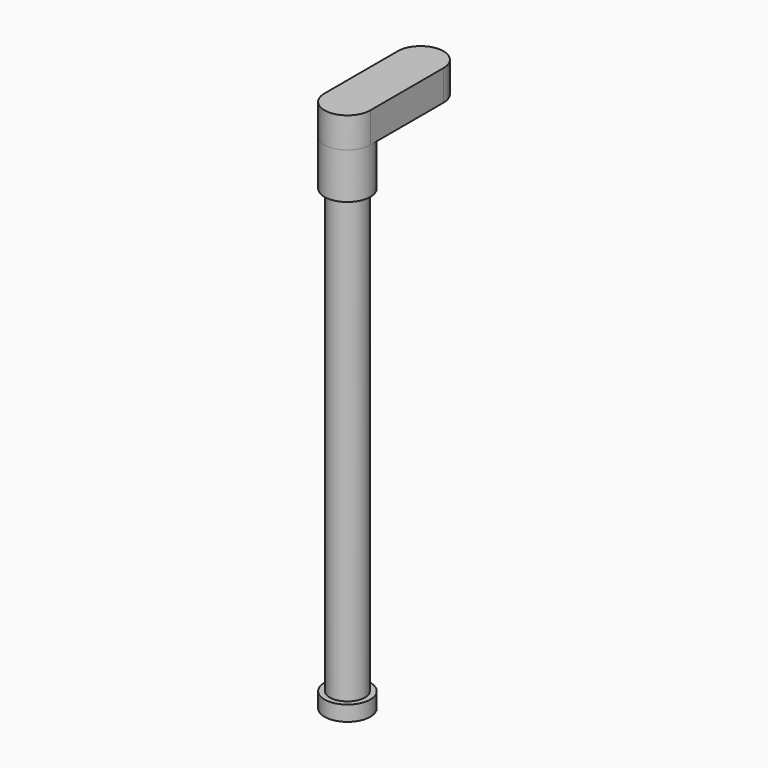
from build123d import *

# Parameters (mm, degrees)
F0_R     = 2.921
F1_DEPTH = 73.66
F2_R     = 3.81
F2_R_2   = 2.921
F3_DEPTH = 2.54
F4_R     = 3.81
F5_DEPTH = 7.62
F7_DEPTH = 5.08


with BuildPart() as f1:
    # F0 (on Top) → F1 (new body)
    with BuildSketch(Plane.XY):
        Circle(F0_R)
    extrude(amount=F1_DEPTH)

    # F2 (on face) → F3 (join)
    with BuildSketch(Plane(origin=(0, 0, 0), x_dir=(1, 0, 0), z_dir=(0, 0, -1))):
        Circle(F2_R)
        Circle(F2_R_2, mode=Mode.SUBTRACT)
        Circle(F2_R_2)
    extrude(amount=F3_DEPTH)

    # F4 (on face) → F5 (join)
    with BuildSketch(Plane.XY.offset(73.66)):
        Circle(F4_R)
    extrude(amount=F5_DEPTH)

    # F6 (on face) → F7 (join)
    with BuildSketch(Plane.XY.offset(81.28)):
        with BuildLine():
            ThreePointArc((-3.81, 0), (0, 3.81), (3.81, 0))
            Line((3.81, 0), (3.81, 15.24))
            ThreePointArc((3.81, 15.24), (0, 11.43), (-3.81, 15.24))
            Line((-3.81, 15.24), (-3.81, 0))
        make_face()
        with BuildLine():
            Line((-3.81, 0), (3.81, 0))
            ThreePointArc((3.81, 0), (0, 3.81), (-3.81, 0))
        make_face()
        with BuildLine():
            ThreePointArc((-3.81, 0), (0, -3.81), (3.81, 0))
            Line((3.81, 0), (-3.81, 0))
        make_face()
        with BuildLine():
            Line((-3.81, 15.24), (3.81, 15.24))
            ThreePointArc((3.81, 15.24), (0, 19.05), (-3.81, 15.24))
        make_face()
        with BuildLine():
            ThreePointArc((-3.81, 15.24), (0, 11.43), (3.81, 15.24))
            Line((3.81, 15.24), (-3.81, 15.24))
        make_face()
    extrude(amount=F7_DEPTH)


solid = f1.part
